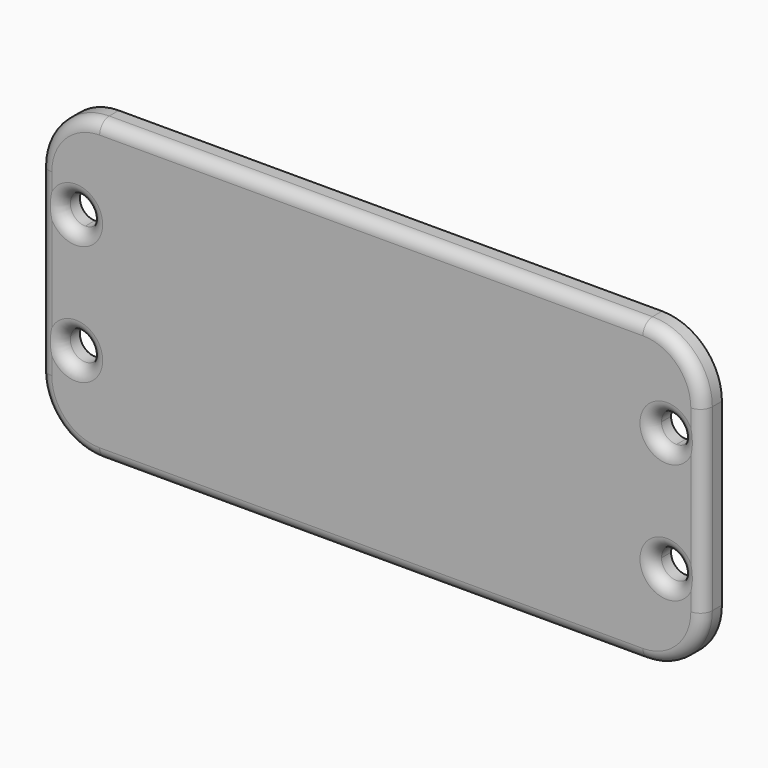
from build123d import *

# Parameters (mm, degrees)
F0_W         = 41
F0_H         = 10
F1_DEPTH     = 2
F2_DEPTH     = 1
F3_T1_DEPTH  = 45.4
F3_T3_DEPTH  = 15
F3_T6_ANGLE  = 90
F3_T8_ANGLE  = 90
F3_T10_ANGLE = 90
F3_T12_ANGLE = 90


# Not quite as in the source:
# - a fillet or chamfer that OpenCascade refuses, or shapes differently, is made with other operations: its cross-section is extruded or revolved along the edge and cut away or added


with BuildPart() as f1:
    # F0 (on Front) → F1 (new body)
    with BuildSketch(Plane.XZ):
        with BuildLine():
            Line((43.4, 23), (-2, 23))
            ThreePointArc((-2, 23), (-5.5355339059, 21.5355339059), (-7, 18))
            Line((-7, 18), (-7, 3))
            ThreePointArc((-7, 3), (-5.5355339059, -0.5355339059), (-2, -2))
            Line((-2, -2), (43.4, -2))
            ThreePointArc((43.4, -2), (46.9355339059, -0.5355339059), (48.4, 3))
            Line((48.4, 3), (48.4, 18))
            ThreePointArc((48.4, 18), (46.9355339059, 21.5355339059), (43.4, 23))
        make_face()
        with BuildLine():
            Line((36, 0), (5, 0))
            ThreePointArc((5, 0), (1.4644660941, 1.4644660941), (0, 5))
            Line((0, 5), (0, 5.5))
            Line((0, 5.5), (-2.75, 5.5))
            ThreePointArc((-2.75, 5.5), (-4.8838834765, 4.6161165235), (-4, 6.75))
            Line((-4, 6.75), (-4, 14.25))
            ThreePointArc((-4, 14.25), (-4.8838834765, 16.3838834765), (-2.75, 15.5))
            Line((-2.75, 15.5), (0, 15.5))
            Line((0, 15.5), (0, 16))
            ThreePointArc((0, 16), (1.4644660941, 19.5355339059), (5, 21))
            Line((5, 21), (36, 21))
            ThreePointArc((36, 21), (39.5355339059, 19.5355339059), (41, 16))
            Line((41, 16), (41, 15.5))
            Line((41, 15.5), (44.15, 15.5))
            ThreePointArc((44.15, 15.5), (45.4, 16.75), (46.65, 15.5))
            ThreePointArc((46.65, 15.5), (46.2838834765, 14.6161165235), (45.4, 14.25))
            Line((45.4, 14.25), (45.4, 6.75))
            ThreePointArc((45.4, 6.75), (46.2838834765, 6.3838834765), (46.65, 5.5))
            ThreePointArc((46.65, 5.5), (45.4, 4.25), (44.15, 5.5))
            Line((44.15, 5.5), (41, 5.5))
            Line((41, 5.5), (41, 5))
            ThreePointArc((41, 5), (39.5355339059, 1.4644660941), (36, 0))
        make_face(mode=Mode.SUBTRACT)
        with BuildLine():
            Line((0, 16), (0, 15.5))
            Line((0, 15.5), (41, 15.5))
            Line((41, 15.5), (41, 16))
            ThreePointArc((41, 16), (39.5355339059, 19.5355339059), (36, 21))
            Line((36, 21), (5, 21))
            ThreePointArc((5, 21), (1.4644660941, 19.5355339059), (0, 16))
        make_face()
        with BuildLine():
            Line((-2.75, 5.5), (0, 5.5))
            Line((0, 5.5), (0, 15.5))
            Line((0, 15.5), (-2.75, 15.5))
            ThreePointArc((-2.75, 15.5), (-3.1161165235, 14.6161165235), (-4, 14.25))
            Line((-4, 14.25), (-4, 6.75))
            ThreePointArc((-4, 6.75), (-3.1161165235, 6.3838834765), (-2.75, 5.5))
        make_face()
        with Locations((20.5, 10.5)):
            Rectangle(F0_W, F0_H)
        with BuildLine():
            Line((41, 15.5), (41, 5.5))
            Line((41, 5.5), (44.15, 5.5))
            ThreePointArc((44.15, 5.5), (44.5161165235, 6.3838834765), (45.4, 6.75))
            Line((45.4, 6.75), (45.4, 14.25))
            ThreePointArc((45.4, 14.25), (44.5161165235, 14.6161165235), (44.15, 15.5))
            Line((44.15, 15.5), (41, 15.5))
        make_face()
        with BuildLine():
            ThreePointArc((0, 5), (1.4644660941, 1.4644660941), (5, 0))
            Line((5, 0), (36, 0))
            ThreePointArc((36, 0), (39.5355339059, 1.4644660941), (41, 5))
            Line((41, 5), (41, 5.5))
            Line((41, 5.5), (0, 5.5))
            Line((0, 5.5), (0, 5))
        make_face()
    extrude(amount=F1_DEPTH)

    # F0 (on Front) → F2 (join)
    with BuildSketch(Plane.XZ):
        with BuildLine():
            Line((0, 16), (0, 15.5))
            Line((0, 15.5), (41, 15.5))
            Line((41, 15.5), (41, 16))
            ThreePointArc((41, 16), (39.5355339059, 19.5355339059), (36, 21))
            Line((36, 21), (5, 21))
            ThreePointArc((5, 21), (1.4644660941, 19.5355339059), (0, 16))
        make_face()
        with Locations((20.5, 10.5)):
            Rectangle(F0_W, F0_H)
        with BuildLine():
            ThreePointArc((0, 5), (1.4644660941, 1.4644660941), (5, 0))
            Line((5, 0), (36, 0))
            ThreePointArc((36, 0), (39.5355339059, 1.4644660941), (41, 5))
            Line((41, 5), (41, 5.5))
            Line((41, 5.5), (0, 5.5))
            Line((0, 5.5), (0, 5))
        make_face()
    extrude(amount=-F2_DEPTH)

    # F3: fillet of radius 1 on 12 edges, made by hand

    # F3_s2 → F3_t1 (cut)
    with BuildSketch(Plane.YZ.offset(-2)):
        with BuildLine():
            ThreePointArc((-1, 23), (-1.7071067812, 22.7071067812), (-2, 22))
            Line((-2, 22), (-2, 23))
            Line((-2, 23), (-1, 23))
        make_face()
        with BuildLine():
            ThreePointArc((-2, -1), (-1.7071067812, -1.7071067812), (-1, -2))
            Line((-1, -2), (-2, -2))
            Line((-2, -2), (-2, -1))
        make_face()
    extrude(amount=F3_T1_DEPTH, mode=Mode.SUBTRACT)

    # F3_s4 → F3_t3 (cut)
    with BuildSketch(Plane.XY.offset(3)):
        with BuildLine():
            ThreePointArc((-6, -2), (-6.7071067812, -1.7071067812), (-7, -1))
            Line((-7, -1), (-7, -2))
            Line((-7, -2), (-6, -2))
        make_face()
        with BuildLine():
            ThreePointArc((47.4, -2), (48.1071067812, -1.7071067812), (48.4, -1))
            Line((48.4, -1), (48.4, -2))
            Line((48.4, -2), (47.4, -2))
        make_face()
    extrude(amount=F3_T3_DEPTH, mode=Mode.SUBTRACT)

    # F3_s5 → F3_t6 (revolve, cut)
    with BuildSketch(Plane.YZ.offset(-2)):
        with BuildLine():
            ThreePointArc((-1, 23), (-1.7071067812, 22.7071067812), (-2, 22))
            Line((-2, 22), (-2, 23))
            Line((-2, 23), (-1, 23))
        make_face()
    revolve(axis=Axis((-2, -2, 18), (0, -1, 0)), revolution_arc=F3_T6_ANGLE, mode=Mode.SUBTRACT)

    # F3_s7 → F3_t8 (revolve, cut)
    with BuildSketch(Plane.XY.offset(3)):
        with BuildLine():
            ThreePointArc((-6, -2), (-6.7071067812, -1.7071067812), (-7, -1))
            Line((-7, -1), (-7, -2))
            Line((-7, -2), (-6, -2))
        make_face()
    revolve(axis=Axis((-2, -2, 3), (0, -1, 0)), revolution_arc=F3_T8_ANGLE, mode=Mode.SUBTRACT)

    # F3_s9 → F3_t10 (revolve, cut)
    with BuildSketch(Plane.YZ.offset(43.4)):
        with BuildLine():
            ThreePointArc((-2, -1), (-1.7071067812, -1.7071067812), (-1, -2))
            Line((-1, -2), (-2, -2))
            Line((-2, -2), (-2, -1))
        make_face()
    revolve(axis=Axis((43.4, -2, 3), (0, -1, 0)), revolution_arc=F3_T10_ANGLE, mode=Mode.SUBTRACT)

    # F3_s11 → F3_t12 (revolve, cut)
    with BuildSketch(Plane.XY.offset(18)):
        with BuildLine():
            ThreePointArc((48.4, -1), (48.1071067812, -1.7071067812), (47.4, -2))
            Line((47.4, -2), (48.4, -2))
            Line((48.4, -2), (48.4, -1))
        make_face()
    revolve(axis=Axis((43.4, -2, 18), (0, -1, 0)), revolution_arc=F3_T12_ANGLE, mode=Mode.SUBTRACT)

    # F3_s13 → F3_t14 (revolve, cut)
    with BuildSketch(Plane.YZ.offset(-4)):
        with BuildLine():
            ThreePointArc((-2, 7.75), (-1.7071067812, 7.0428932188), (-1, 6.75))
            Line((-1, 6.75), (-2, 6.75))
            Line((-2, 6.75), (-2, 7.75))
        make_face()
    revolve(axis=Axis((-4, -2, 5.5), (0, 1, 0)), mode=Mode.SUBTRACT)

    # F3_s15 → F3_t16 (revolve, cut)
    with BuildSketch(Plane.XY.offset(15.5)):
        with BuildLine():
            ThreePointArc((-1.75, -2), (-2.4571067812, -1.7071067812), (-2.75, -1))
            Line((-2.75, -1), (-2.75, -2))
            Line((-2.75, -2), (-1.75, -2))
        make_face()
    revolve(axis=Axis((-4, -2, 15.5), (0, 1, 0)), mode=Mode.SUBTRACT)

    # F3_s17 → F3_t18 (revolve, cut)
    with BuildSketch(Plane.XY.offset(5.5)):
        with BuildLine():
            ThreePointArc((43.15, -2), (43.8571067812, -1.7071067812), (44.15, -1))
            Line((44.15, -1), (44.15, -2))
            Line((44.15, -2), (43.15, -2))
        make_face()
    revolve(axis=Axis((45.4, -2, 5.5), (0, 1, 0)), mode=Mode.SUBTRACT)

    # F3_s19 → F3_t20 (revolve, cut)
    with BuildSketch(Plane.YZ.offset(45.4)):
        with BuildLine():
            ThreePointArc((-2, 13.25), (-1.7071067812, 13.9571067812), (-1, 14.25))
            Line((-1, 14.25), (-2, 14.25))
            Line((-2, 14.25), (-2, 13.25))
        make_face()
    revolve(axis=Axis((45.4, -2, 15.5), (0, 1, 0)), mode=Mode.SUBTRACT)


solid = f1.part
